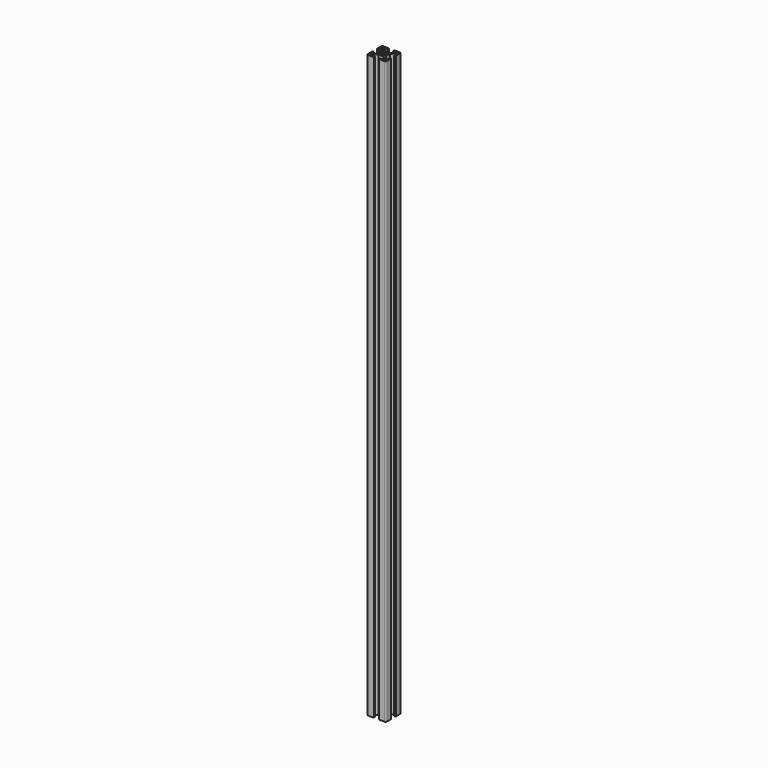
from build123d import *

# Parameters (mm, degrees)
F1_DEPTH = 914.4


# Not quite as in the source:
# - ends of sketch curves that miss each other by under 0.0002 mm in the source are joined


with BuildPart() as f1:
    # F0 (on Top) → F1 (new body)
    with BuildSketch(Plane.XY):
        with BuildLine():
            Line((-10.053123, -8.25), (-12.8, -8.25))
            Line((-12.8, -8.25), (-12.800036, -4.05))
            Line((-12.800036, -4.05), (-14.5, -4.05))
            Line((-14.5, -4.05), (-14.5, -4.55))
            Line((-14.5, -4.55), (-15, -4.55))
            Line((-15, -4.55), (-15, -13))
            ThreePointArc((-15, -13), (-14.4142135624, -14.4142135624), (-13, -15))
            Line((-13, -15), (-4.55, -15))
            Line((-4.55, -15), (-4.55, -14.5))
            Line((-4.55, -14.5), (-4.05, -14.5))
            Line((-4.05, -14.5), (-4.05, -12.800036))
            Line((-4.05, -12.800036), (-8.25, -12.8))
            Line((-8.25, -12.8), (-8.25, -10.053123))
            Line((-8.25, -10.053123), (-4.196877, -6))
            Line((-4.196877, -6), (4.196877, -6))
            Line((4.196877, -6), (8.25, -10.053123))
            Line((8.25, -10.053123), (8.25, -12.8))
            Line((8.25, -12.8), (4.05, -12.800036))
            Line((4.05, -12.800036), (4.05, -14.5))
            Line((4.05, -14.5), (4.55, -14.5))
            Line((4.55, -14.5), (4.55, -15))
            Line((4.55, -15), (13, -15))
            ThreePointArc((13, -15), (14.4142135624, -14.4142135624), (15, -13))
            Line((15, -13), (15, -4.55))
            Line((15, -4.55), (14.5, -4.55))
            Line((14.5, -4.55), (14.5, -4.05))
            Line((14.5, -4.05), (12.800036, -4.05))
            Line((12.800036, -4.05), (12.8, -8.25))
            Line((12.8, -8.25), (10.053123, -8.25))
            Line((10.053123, -8.25), (6, -4.196877))
            Line((6, -4.196877), (6, 4.196877))
            Line((6, 4.196877), (10.053123, 8.25))
            Line((10.053123, 8.25), (12.8, 8.25))
            Line((12.8, 8.25), (12.800036, 4.05))
            Line((12.800036, 4.05), (14.5, 4.05))
            Line((14.5, 4.05), (14.5, 4.55))
            Line((14.5, 4.55), (15, 4.55))
            Line((15, 4.55), (15, 13))
            ThreePointArc((15, 13), (14.4142135624, 14.4142135624), (13, 15))
            Line((13, 15), (4.55, 15))
            Line((4.55, 15), (4.55, 14.5))
            Line((4.55, 14.5), (4.05, 14.5))
            Line((4.05, 14.5), (4.05, 12.800036))
            Line((4.05, 12.800036), (8.25, 12.8))
            Line((8.25, 12.8), (8.25, 10.053123))
            Line((8.25, 10.053123), (4.196877, 6))
            Line((4.196877, 6), (-4.196877, 6))
            Line((-4.196877, 6), (-8.25, 10.053123))
            Line((-8.25, 10.053123), (-8.25, 12.8))
            Line((-8.25, 12.8), (-4.05, 12.800036))
            Line((-4.05, 12.800036), (-4.05, 14.5))
            Line((-4.05, 14.5), (-4.55, 14.5))
            Line((-4.55, 14.5), (-4.55, 15))
            Line((-4.55, 15), (-13, 15))
            ThreePointArc((-13, 15), (-14.4142135624, 14.4142135624), (-15, 13))
            Line((-15, 13), (-15, 4.55))
            Line((-15, 4.55), (-14.5, 4.55))
            Line((-14.5, 4.55), (-14.5, 4.05))
            Line((-14.5, 4.05), (-12.800036, 4.05))
            Line((-12.800036, 4.05), (-12.8, 8.25))
            Line((-12.8, 8.25), (-10.053123, 8.25))
            Line((-10.053123, 8.25), (-6, 4.196877))
            Line((-6, 4.196877), (-6, -4.196877))
            Line((-6, -4.196877), (-10.053123, -8.25))
        make_face()
        with BuildLine():
            Line((-9.7, -13.85), (-12.85, -13.85))
            ThreePointArc((-12.85, -13.85), (-13.5571067812, -13.5571067812), (-13.85, -12.85))
            Line((-13.85, -12.85), (-13.85, -9.7))
            Line((-13.85, -9.7), (-9.7, -9.7))
            Line((-9.7, -9.7), (-9.7, -13.85))
        make_face(mode=Mode.SUBTRACT)
        with BuildLine():
            Line((12.85, -13.85), (9.7, -13.85))
            Line((9.7, -13.85), (9.7, -9.7))
            Line((9.7, -9.7), (13.85, -9.7))
            Line((13.85, -9.7), (13.85, -12.85))
            ThreePointArc((13.85, -12.85), (13.5571067812, -13.5571067812), (12.85, -13.85))
        make_face(mode=Mode.SUBTRACT)
        with BuildLine():
            Line((-9.7, 9.7), (-13.85, 9.7))
            Line((-13.85, 9.7), (-13.85, 12.85))
            ThreePointArc((-13.85, 12.85), (-13.5571067812, 13.5571067812), (-12.85, 13.85))
            Line((-12.85, 13.85), (-9.7, 13.85))
            Line((-9.7, 13.85), (-9.7, 9.7))
        make_face(mode=Mode.SUBTRACT)
        with BuildLine():
            Line((3.272394, -1.616767), (4.590523, -3.187652))
            Line((4.590523, -3.187652), (3.187652, -4.590523))
            Line((3.187652, -4.590523), (1.616767, -3.272394))
            ThreePointArc((1.616767, -3.272394), (0, -3.65), (-1.6167671199, -3.2723942427))
            Line((-1.6167671199, -3.2723942427), (-3.187652, -4.590523))
            Line((-3.187652, -4.590523), (-4.590523, -3.187652))
            Line((-4.590523, -3.187652), (-3.272394, -1.616767))
            ThreePointArc((-3.272394, -1.616767), (-3.65, 0), (-3.2723942427, 1.6167671199))
            Line((-3.2723942427, 1.6167671199), (-4.590523, 3.187652))
            Line((-4.590523, 3.187652), (-3.187652, 4.590523))
            Line((-3.187652, 4.590523), (-1.616767, 3.272394))
            ThreePointArc((-1.616767, 3.272394), (0, 3.65), (1.6167671199, 3.2723942427))
            Line((1.6167671199, 3.2723942427), (3.187652, 4.590523))
            Line((3.187652, 4.590523), (4.590523, 3.187652))
            Line((4.590523, 3.187652), (3.272394, 1.616767))
            ThreePointArc((3.272394, 1.616767), (3.65, 0), (3.272394, -1.616767))
        make_face(mode=Mode.SUBTRACT)
        with BuildLine():
            Line((13.85, 9.7), (9.7, 9.7))
            Line((9.7, 9.7), (9.7, 13.85))
            Line((9.7, 13.85), (12.85, 13.85))
            ThreePointArc((12.85, 13.85), (13.5571067812, 13.5571067812), (13.85, 12.85))
            Line((13.85, 12.85), (13.85, 9.7))
        make_face(mode=Mode.SUBTRACT)
    extrude(amount=F1_DEPTH)


solid = f1.part
